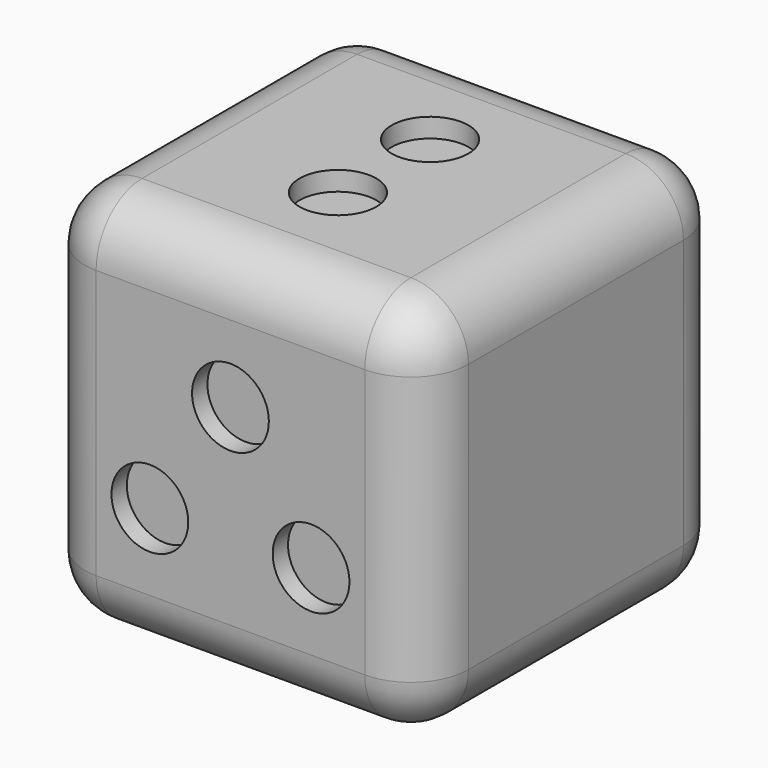
from build123d import *

# Parameters (mm, degrees)
F0_W      = 100
F0_H      = 100
F1_DEPTH  = 100
F2_F1_R   = 15
F2_F2_R   = 15
F2_F3_R   = 15
F2_F4_R   = 15
F2_F5_R   = 15
F4_R      = 10
F5_DEPTH  = 5
F7_R      = 10
F8_DEPTH  = 5
F9_R      = 10
F10_DEPTH = 5


# Not quite as in the source:
# - a feature of the source that left no trace in its solid (it failed there, or was rolled back) is left out


with BuildPart() as f1:
    # F0 (on Top) → F1 (new body)
    with BuildSketch(Plane.XY):
        Rectangle(F0_W, F0_H)
    extrude(amount=F1_DEPTH)

    # F2: fillet of radius 15 on 7 edges, made by hand

    # F2_f1
    f2_f1_edges = [f1.edges().sort_by_distance(p)[0] for p in [
        (50, 50, 50),
    ]]
    fillet(f2_f1_edges, radius=F2_F1_R)

    # F2_f2
    f2_f2_edges = [f1.edges().sort_by_distance(p)[0] for p in [
        (-50, 50, 50),
    ]]
    fillet(f2_f2_edges, radius=F2_F2_R)

    # F2_f3
    f2_f3_edges = [f1.edges().sort_by_distance(p)[0] for p in [
        (0, 50, 100),
    ]]
    fillet(f2_f3_edges, radius=F2_F3_R)

    # F2_f4
    f2_f4_edges = [f1.edges().sort_by_distance(p)[0] for p in [
        (-50, -50, 42.5),
    ]]
    fillet(f2_f4_edges, radius=F2_F4_R)

    # F2_f5
    f2_f5_edges = [f1.edges().sort_by_distance(p)[0] for p in [
        (-50, 0, 0),
    ]]
    fillet(f2_f5_edges, radius=F2_F5_R)

    # F4 (on Top) → F5 (cut)
    with BuildSketch(Plane.XY):
        Circle(F4_R)
    extrude(amount=F5_DEPTH, mode=Mode.SUBTRACT)

    # F7 (on face) → F8 (cut)
    with BuildSketch(Plane.XY.offset(100)):
        with Locations((0, -15)):
            Circle(F7_R)
        with Locations((0, 15)):
            Circle(F7_R)
    extrude(amount=-F8_DEPTH, mode=Mode.SUBTRACT)

    # F9 (on face) → F10 (cut)
    with BuildSketch(Plane.XZ.offset(50)):
        with Locations((0, 65)):
            Circle(F9_R)
        with Locations((-21, 35)):
            Circle(F9_R)
        with Locations((21, 35)):
            Circle(F9_R)
    extrude(amount=-F10_DEPTH, mode=Mode.SUBTRACT)


solid = f1.part
